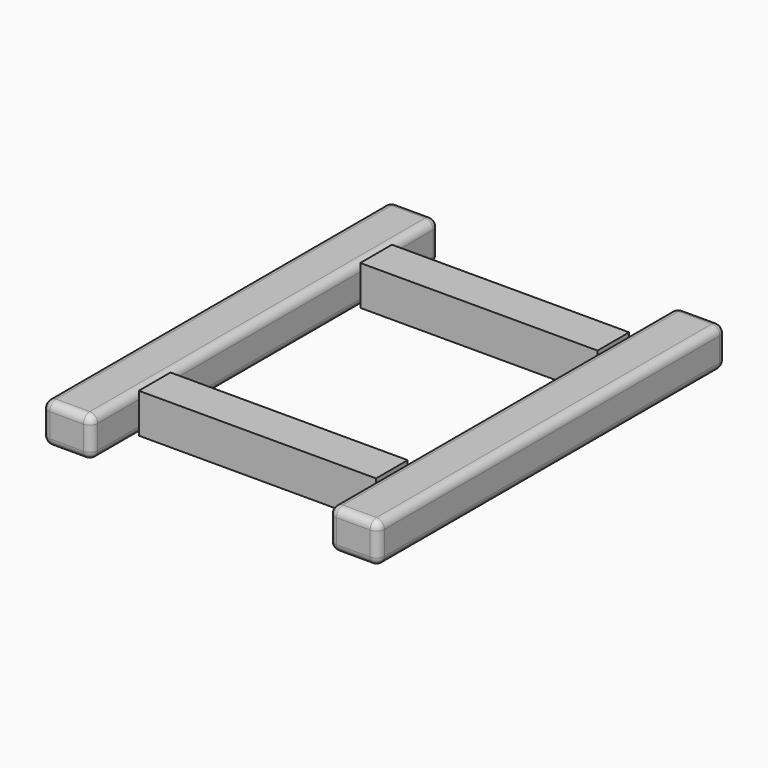
from build123d import *

# Parameters (mm, degrees)
F1_DEPTH = 25.4
F3_W     = 25.4
F3_H     = 25.4
F4_DEPTH = 152.4
F6_R     = 3.175
F7_DEPTH = 76.2
F8_R     = 5.08
F8_2_R   = 5.08
F9_R     = 5.08
F9_2_R   = 5.08


with BuildPart() as f1:
    # F0 (on Top) → F1 (new body)
    with BuildSketch(Plane.XY):
        Polygon((-76.2, 139.7), (-107.95, 139.7), (-107.95, -139.7), (-76.2, -139.7), (-76.2, 0), align=None)
    extrude(amount=F1_DEPTH)


with BuildPart() as f2_1:
    # F2: instance of F1
    add(f1.part.mirror(Plane.YZ))

    # F8#2
    f8_2_edges = [f2_1.edges().sort_by_distance(p)[0] for p in [
        (76.2, -139.7, 12.7),
        (107.95, -139.7, 12.7),
        (107.95, 139.7, 12.7),
        (76.2, 139.7, 12.7),
    ]]
    fillet(f8_2_edges, radius=F8_2_R)

    # F9#2
    f9_2_edges = [f2_1.edges().sort_by_distance(p)[0] for p in [
        (107.95, 0, 25.4),
        (107.95, 0, 0),
        (92.075, 139.7, 0),
        (92.075, 139.7, 25.4),
        (77.687898, 138.212102, 0),
        (106.462102, 138.212102, 0),
        (77.687898, -138.212102, 0),
        (106.462102, -138.212102, 0),
        (92.075, -139.7, 0),
        (77.687898, 138.212102, 25.4),
        (106.462102, 138.212102, 25.4),
        (77.687898, -138.212102, 25.4),
        (106.462102, -138.212102, 25.4),
        (92.075, -139.7, 25.4),
    ]]
    fillet(f9_2_edges, radius=F9_2_R)


with BuildPart() as f4:
    # F3 (on face) → F4 (new body, through all)
    with BuildSketch(Plane.YZ.offset(-76.2)):
        with Locations((-88.9, 12.7)):
            Rectangle(F3_W, F3_H)
    extrude(amount=F4_DEPTH)


with BuildPart() as f5_1:
    # F5: instance of F4
    add(f4.part.mirror(Plane.XZ))


with BuildPart() as f1_1:
    add(f1.part)

    # F6 (on face) → F7 (cut)
    with BuildSketch(Plane(origin=(-107.95, 0, 0), x_dir=(0, -1, 0), z_dir=(-1, 0, 0))):
        with Locations((94.1916666667, 12.7)):
            Circle(F6_R)
        with Locations((83.6083333333, 12.7)):
            Circle(F6_R)
        with Locations((-83.6083333333, 12.7)):
            Circle(F6_R)
        with Locations((-94.1916666667, 12.7)):
            Circle(F6_R)
    extrude(amount=-F7_DEPTH, mode=Mode.SUBTRACT)

    # F8
    f8_edges = [f1_1.edges().sort_by_distance(p)[0] for p in [
        (-107.95, -139.7, 12.7),
        (-76.2, -139.7, 12.7),
        (-76.2, 139.7, 12.7),
        (-107.95, 139.7, 12.7),
    ]]
    fillet(f8_edges, radius=F8_R)

    # F9
    f9_edges = [f1_1.edges().sort_by_distance(p)[0] for p in [
        (-107.95, 0, 25.4),
        (-107.95, 0, 0),
        (-92.075, 139.7, 0),
        (-92.075, 139.7, 25.4),
        (-77.687898, 138.212102, 0),
        (-106.462102, 138.212102, 0),
        (-77.687898, -138.212102, 0),
        (-106.462102, -138.212102, 0),
        (-92.075, -139.7, 0),
        (-77.687898, 138.212102, 25.4),
        (-106.462102, 138.212102, 25.4),
        (-77.687898, -138.212102, 25.4),
        (-106.462102, -138.212102, 25.4),
        (-92.075, -139.7, 25.4),
    ]]
    fillet(f9_edges, radius=F9_R)


solid = Compound([f2_1.part, f4.part, f5_1.part, f1_1.part])
